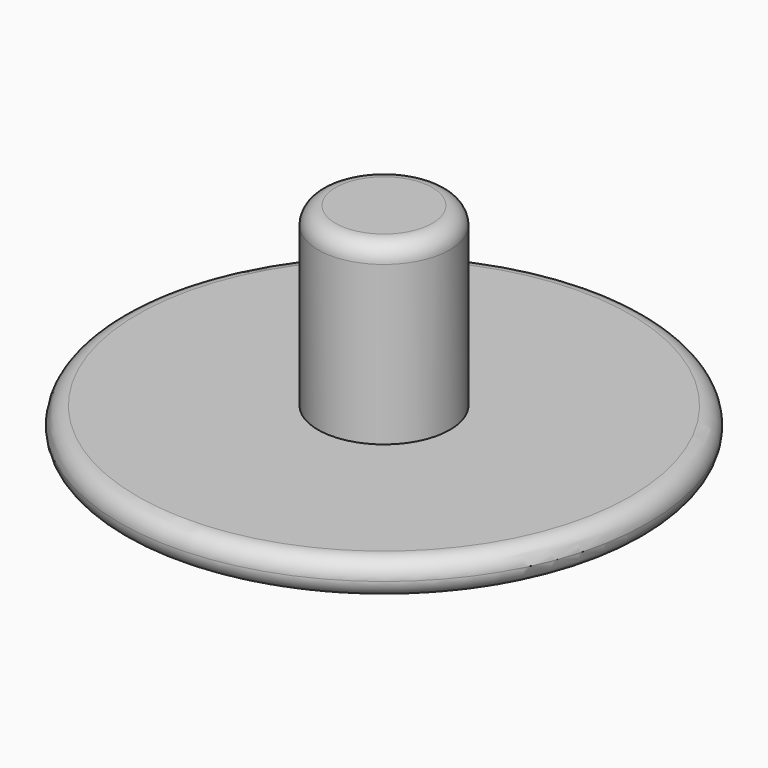
from build123d import *

# Parameters (mm, degrees)
F0_R     = 15
F1_DEPTH = 2
F2_R     = 3.75
F3_DEPTH = 10
F4_R     = 0.99999


# Not quite as in the source:
# - a fillet or chamfer is up to 0.001 mm smaller than in the source, because OpenCascade refuses the exact size


with BuildPart() as f1:
    # F0 (on Top) → F1 (new body)
    with BuildSketch(Plane.XY):
        Circle(F0_R)
    extrude(amount=F1_DEPTH)

    # F2 (on face) → F3 (join)
    with BuildSketch(Plane.XY.offset(2)):
        Circle(F2_R)
    extrude(amount=F3_DEPTH)

    # F4 (radius 1 in the source; OpenCascade refuses exactly that, so slightly less here)
    f4_edges = [f1.edges().sort_by_distance(p)[0] for p in [
        (-3.75, 0, 12),
        (15, 0, 1),
        (-15, 0, 0),
        (-15, 0, 2),
    ]]
    fillet(f4_edges, radius=F4_R)


solid = f1.part
